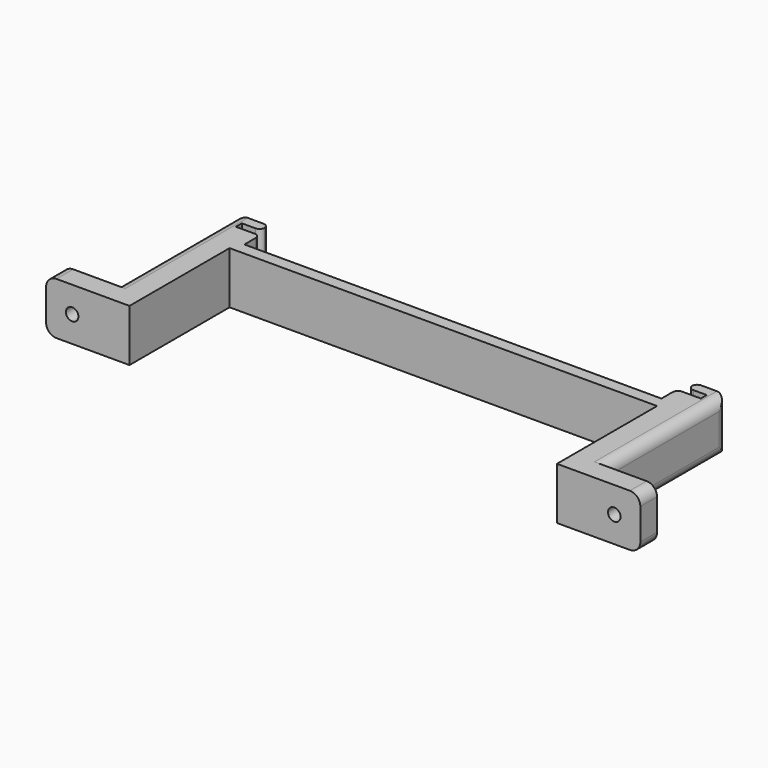
from build123d import *

# Parameters (mm, degrees)
F0_W        = 7.62
F0_H        = 5.08
F0_W_2      = 12.7
F0_W_3      = 1.27
F0_H_2      = 4.6902727336
F0_H_3      = 2.9297272664
F0_W_4      = 101.6
F1_DEPTH    = 12.7
F2_T1_DEPTH = 19.05
F3_R        = 1.524
F4_DEPTH    = 25.4
F5_R        = 2.54


# Not quite as in the source:
# - a fillet or chamfer that OpenCascade refuses, or shapes differently, is made with other operations: its cross-section is extruded or revolved along the edge and cut away or added


with BuildPart() as f1:
    # F0 (on Top) → F1 (new body)
    with BuildSketch(Plane.XY):
        Polygon((-47.2217758975, 22.7881683916), (-54.8417758975, 22.7881683916), (-54.8417758975, -14.4997123967), (-47.2217758975, -14.4997123967), (-47.2217758975, 10.9002876033), (-47.2217758975, 13.8300148697), (-47.2217758975, 18.5202876033), (-51.7937758975, 18.5202876033), (-51.7937758975, 20.344916165), (-47.2217758975, 20.344916165), align=None)
        with Locations((-51.0317758975, -17.0397123967)):
            Rectangle(F0_W, F0_H)
        with Locations((-61.1917758975, -17.0397123967)):
            Rectangle(F0_W_2, F0_H)
        Polygon((64.5382241025, 22.7881683916), (56.9182241025, 22.7881683916), (56.9182241025, 20.344916165), (61.4902241025, 20.344916165), (61.4902241025, 18.5202876033), (56.9182241025, 18.5202876033), (56.9182241025, 13.8300148697), (56.9182241025, 10.9002876033), (56.9182241025, -14.4997123967), (64.5382241025, -14.4997123967), align=None)
        with Locations((-46.5867758975, 16.1751512365)):
            Rectangle(F0_W_3, F0_H_2)
        with Locations((60.7282241025, -17.0397123967)):
            Rectangle(F0_W, F0_H)
        with Locations((-46.5867758975, 12.3651512365)):
            Rectangle(F0_W_3, F0_H_3)
        with Locations((70.8882241025, -17.0397123967)):
            Rectangle(F0_W_2, F0_H)
        with Locations((56.2832241025, 16.1751512365)):
            Rectangle(F0_W_3, F0_H_2)
        with Locations((56.2832241025, 12.3651512365)):
            Rectangle(F0_W_3, F0_H_3)
        with Locations((4.8482241025, 12.3651512365)):
            Rectangle(F0_W_4, F0_H_3)
    extrude(amount=F1_DEPTH)

    # F2: fillet of radius 1.27 on 6 edges, made by hand

    # F2_s2 → F2_t1 (cut)
    with BuildSketch(Plane.XY.offset(-3.175)):
        with BuildLine():
            ThreePointArc((-48.4917758975, 22.7881683916), (-47.5937502854, 22.4161940037), (-47.2217758975, 21.5181683916))
            Line((-47.2217758975, 21.5181683916), (-47.2217758975, 22.7881683916))
            Line((-47.2217758975, 22.7881683916), (-48.4917758975, 22.7881683916))
        make_face()
        with BuildLine():
            ThreePointArc((-45.9517758975, 17.2502876033), (-46.3237502854, 18.1483132154), (-47.2217758975, 18.5202876033))
            Line((-47.2217758975, 18.5202876033), (-45.9517758975, 18.5202876033))
            Line((-45.9517758975, 18.5202876033), (-45.9517758975, 17.2502876033))
        make_face()
        with BuildLine():
            ThreePointArc((-48.4917758975, 20.344916165), (-47.5937502854, 20.7168905529), (-47.2217758975, 21.614916165))
            Line((-47.2217758975, 21.614916165), (-47.2217758975, 20.344916165))
            Line((-47.2217758975, 20.344916165), (-48.4917758975, 20.344916165))
        make_face()
        with BuildLine():
            ThreePointArc((56.9182241025, 18.5202876033), (56.0201984904, 18.1483132154), (55.6482241025, 17.2502876033))
            Line((55.6482241025, 17.2502876033), (55.6482241025, 18.5202876033))
            Line((55.6482241025, 18.5202876033), (56.9182241025, 18.5202876033))
        make_face()
        with BuildLine():
            ThreePointArc((56.9182241025, 21.614916165), (57.2901984904, 20.7168905529), (58.1882241025, 20.344916165))
            Line((58.1882241025, 20.344916165), (56.9182241025, 20.344916165))
            Line((56.9182241025, 20.344916165), (56.9182241025, 21.614916165))
        make_face()
        with BuildLine():
            ThreePointArc((58.1882241025, 22.7881683916), (57.2901984904, 22.4161940037), (56.9182241025, 21.5181683916))
            Line((56.9182241025, 21.5181683916), (56.9182241025, 22.7881683916))
            Line((56.9182241025, 22.7881683916), (58.1882241025, 22.7881683916))
        make_face()
    extrude(amount=F2_T1_DEPTH, mode=Mode.SUBTRACT)

    # F3 (on face) → F4 (cut)
    with BuildSketch(Plane.XZ.offset(19.5797123967)):
        with Locations((-61.1917758975, 6.35)):
            Circle(F3_R)
        with Locations((70.8882241025, 6.35)):
            Circle(F3_R)
    extrude(amount=-F4_DEPTH, mode=Mode.SUBTRACT)

    # F5
    f5_edges = [f1.edges().sort_by_distance(p)[0] for p in [
        (77.238224, -17.039712, 12.7),
        (77.238224, -17.039712, 0),
        (64.538224, 22.788168, 6.35),
        (-54.841776, 22.788168, 6.35),
        (-67.541776, -17.039712, 0),
        (-67.541776, -17.039712, 12.7),
        (-54.841776, 4.144228, 0),
        (-54.841776, 4.144228, 12.7),
        (64.538224, 4.144228, 0),
        (64.538224, 4.144228, 12.7),
    ]]
    fillet(f5_edges, radius=F5_R)


solid = f1.part
